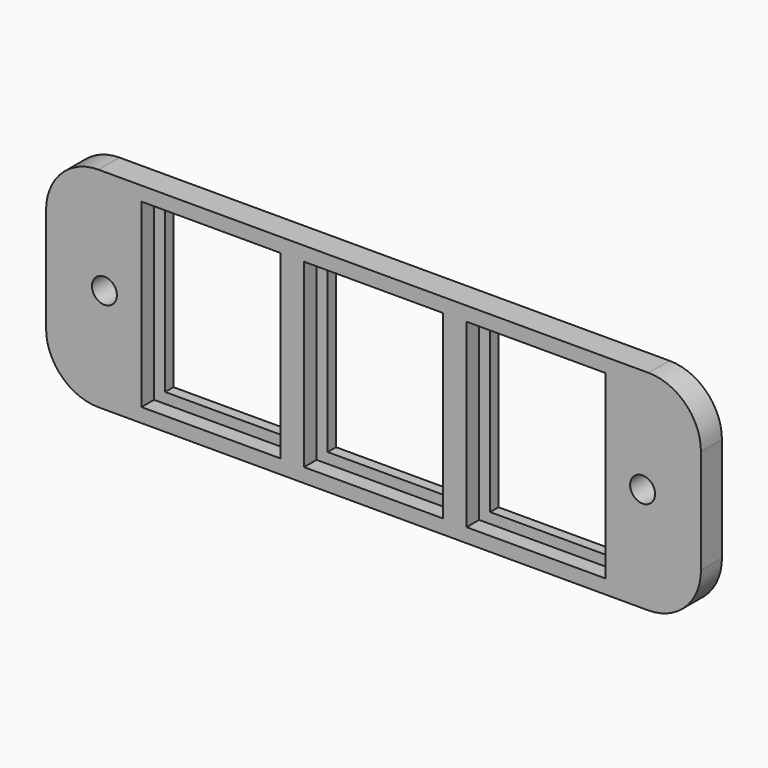
from build123d import *

# Parameters (mm, degrees)
F0_R     = 2.375
F0_W     = 26.5
F0_H     = 34.5
F1_DEPTH = 5
F0_W_2   = 22.3
F0_H_2   = 30.5
F2_DEPTH = 2


# Not quite as in the source:
# - a feature of the source that left no trace in its solid (it failed there, or was rolled back) is left out


with BuildPart() as f1:
    # F0 (on Front) → F1 (new body)
    with BuildSketch(Plane.XZ):
        with BuildLine():
            Line((52.45, 19.95), (-52.45, 19.95))
            ThreePointArc((-52.45, 19.95), (-59.5210678119, 17.0210678119), (-62.45, 9.95))
            Line((-62.45, 9.95), (-62.45, -9.95))
            ThreePointArc((-62.45, -9.95), (-59.5210678119, -17.0210678119), (-52.45, -19.95))
            Line((-52.45, -19.95), (52.45, -19.95))
            ThreePointArc((52.45, -19.95), (59.5210678119, -17.0210678119), (62.45, -9.95))
            Line((62.45, -9.95), (62.45, 9.95))
            ThreePointArc((62.45, 9.95), (59.5210678119, 17.0210678119), (52.45, 19.95))
        make_face()
        with Locations((-51.325, 0)):
            Circle(F0_R, mode=Mode.SUBTRACT)
        with Locations((-31, 0)):
            Rectangle(F0_W, F0_H, mode=Mode.SUBTRACT)
        Rectangle(F0_W, F0_H, mode=Mode.SUBTRACT)
        with Locations((31, 0)):
            Rectangle(F0_W, F0_H, mode=Mode.SUBTRACT)
        with Locations((51.325, 0)):
            Circle(F0_R, mode=Mode.SUBTRACT)
    extrude(amount=F1_DEPTH)

    # F0 (on Front) → F2 (join)
    with BuildSketch(Plane.XZ):
        with Locations((-31, 0)):
            Rectangle(F0_W, F0_H)
        with Locations((-31, 0)):
            Rectangle(F0_W_2, F0_H_2, mode=Mode.SUBTRACT)
        Rectangle(F0_W, F0_H)
        Rectangle(F0_W_2, F0_H_2, mode=Mode.SUBTRACT)
        with Locations((31, 0)):
            Rectangle(F0_W, F0_H)
        with Locations((31, 0)):
            Rectangle(F0_W_2, F0_H_2, mode=Mode.SUBTRACT)
    extrude(amount=F2_DEPTH)


solid = f1.part
